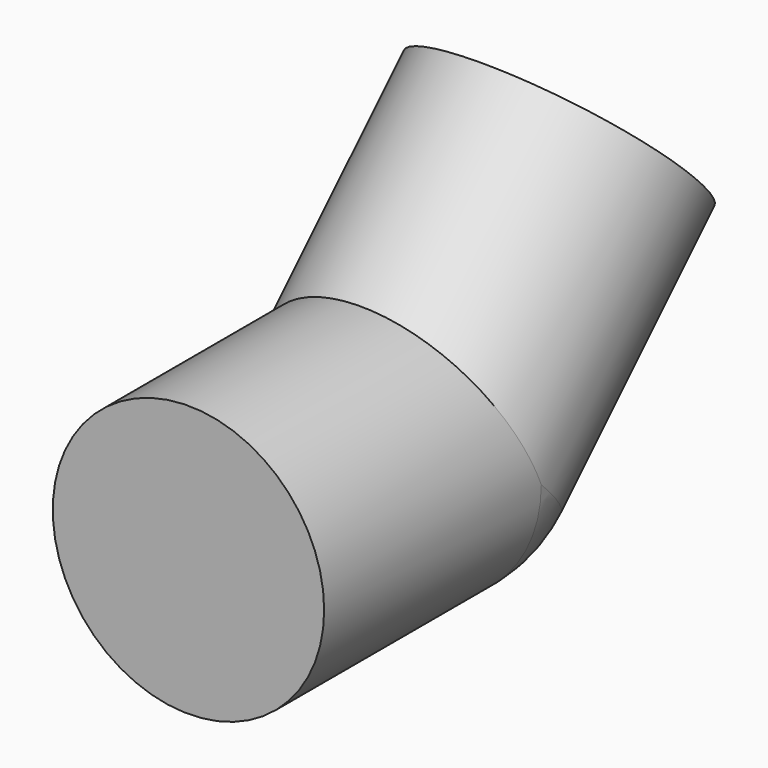
from build123d import *

# Parameters (mm, degrees)
F5_R     = 12.7
F6_DEPTH = 25.4


# Not quite as in the source:
# - a feature of the source that left no trace in its solid (it failed there, or was rolled back) is left out
# - a pattern or mirror of a feature is missing from the dataset's text; its kind, count and spacing are read off the source's solid


with BuildPart() as f4:
    # F3 (on Right) → F4 (revolve)
    with BuildSketch(Plane.YZ):
        with BuildLine():
            Line((0, -12.7), (0, 12.7))
            ThreePointArc((0, 12.7), (-12.7, 0), (0, -12.7))
        make_face()
    revolve(axis=Axis((0, 0, -2.0618988201), (0, 0, -1)))

    # F5 (on Front) → F6 (join)
    with BuildSketch(Plane.XZ):
        Circle(F5_R)
    f6 = extrude(amount=F6_DEPTH)

    # F6_copies: F6 across plane
    add(f6.mirror(Plane(origin=(0, 0, 0), x_dir=(0, -0.3826834324, 0.9238795325), z_dir=(0, 0.9238795325, 0.3826834324))))


solid = f4.part
